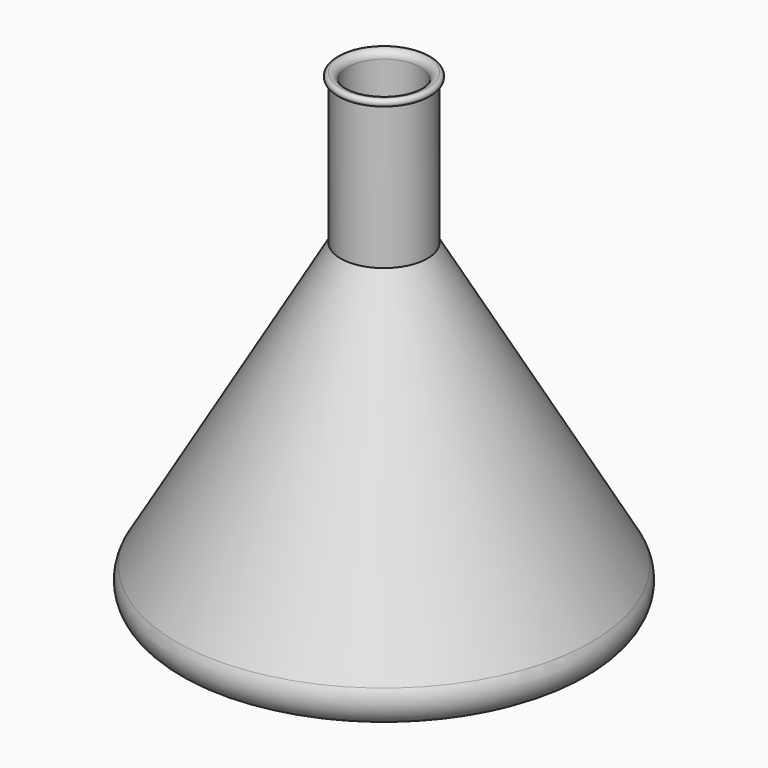
from build123d import *

# Parameters (mm, degrees)
F2_R = 0.99999


# Not quite as in the source:
# - a fillet or chamfer is up to 0.001 mm smaller than in the source, because OpenCascade refuses the exact size


with BuildPart() as f1:
    # F0 (on Front) → F1 (revolve)
    with BuildSketch(Plane.XZ):
        with BuildLine():
            Line((-5, 43.3012701892), (-5, 63.3012701892))
            Line((-5, 63.3012701892), (-5, 64.3012701892))
            Line((-5, 64.3012701892), (-6, 64.3012701892))
            ThreePointArc((-6, 64.3012701892), (-6.5, 63.8012701892), (-6, 63.3012701892))
            Line((-6, 63.3012701892), (-6, 43.5692193817))
            Line((-6, 43.5692193817), (-28.7009618943, 4.25))
            ThreePointArc((-28.7009618943, 4.25), (-28.7009618943, 0.75), (-25.6698729811, -1))
            Line((-25.6698729811, -1), (0, -1))
            Line((0, -1), (0, 0))
            Line((0, 0), (-25.6698729811, 0))
            ThreePointArc((-25.6698729811, 0), (-27.8349364905, 1.25), (-27.8349364905, 3.75))
            Line((-27.8349364905, 3.75), (-5, 43.3012701892))
        make_face()
    revolve(axis=Axis((0, 0, 31.6506350946), (0, 0, 1)))

    # F2 (radius 1 in the source; OpenCascade refuses exactly that, so slightly less here)
    f2_edges = [f1.edges().sort_by_distance(p)[0] for p in [
        (5, 0, 64.30127),
    ]]
    fillet(f2_edges, radius=F2_R)


solid = f1.part
